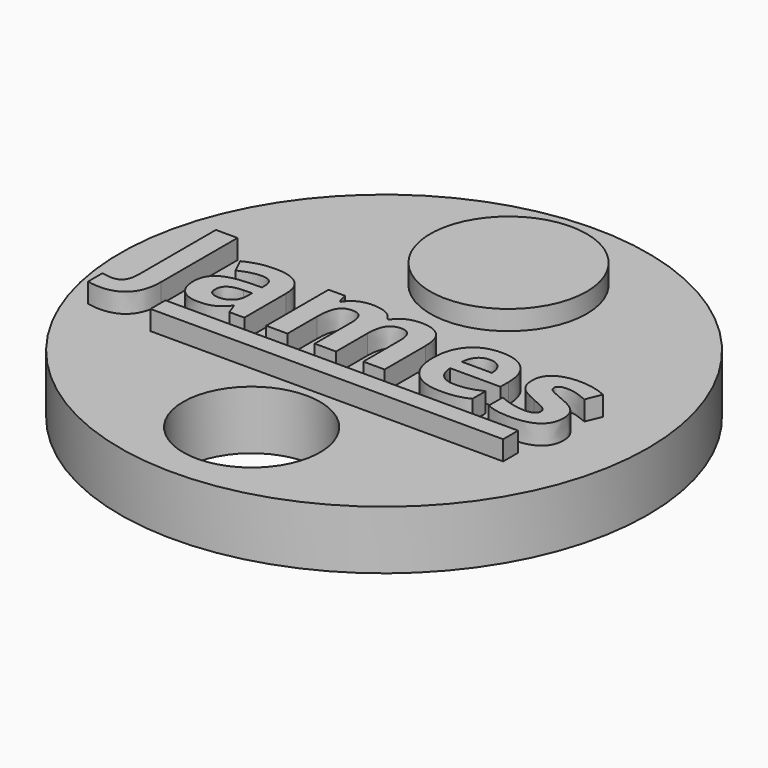
from build123d import *

# Parameters (mm, degrees)
F0_R         = 34.29
F1_DEPTH     = 7.62
F3_DEPTH     = 7.62
F4_TEXT_SIZE = 18.5547053762
F5_DEPTH     = 2.54
F6_R         = 10.16
F7_DEPTH     = 2.54
F10_D        = 15.24
F11_W        = 45.8176825196
F11_H        = 2.4243537337
F12_DEPTH    = 2.54
F15_D        = 17.78


# Not quite as in the source:
# - Text() gives the source's letters only with a copy of the font that has no kerning and outlines rounded to 1/6400 em; it was checked with that copy


with BuildPart() as f1:
    # F0 (on Top) → F1 (new body)
    with BuildSketch(Plane.XY):
        Circle(F0_R)
    extrude(amount=F1_DEPTH)

    # F4 (on face) → F5 (join)
    with BuildSketch(Plane.XY.offset(7.62)):
        with Locations((-28.5104531795, -7.0048975758)):
            Text('James', F4_TEXT_SIZE, font='Open Sans', font_style=FontStyle.BOLD, text_align=(TextAlign.LEFT, TextAlign.BOTTOM))
    extrude(amount=F5_DEPTH)

    # F6 (on face) → F7 (join)
    with BuildSketch(Plane.XY.offset(7.62)):
        with Locations((0.8362137014, 19.1624257714)):
            Circle(F6_R)
    extrude(amount=F7_DEPTH)

    # F11 (on face) → F12 (join)
    with BuildSketch(Plane.XY.offset(7.62)):
        with Locations((1.7281295732, -10.2478833869)):
            Rectangle(F11_W, F11_H)
    extrude(amount=F12_DEPTH)

    # F15 (through all)
    with Locations(Plane.XY.offset(7.62)):
        with Locations((0, -21.506447345)):
            Hole(F15_D / 2)


with BuildPart() as f3:
    # F2 (on face) → F3 (new body)
    with BuildSketch(Plane(origin=(0, 0, 0), x_dir=(1, 0, 0), z_dir=(0, 0, -1))):
        with BuildLine():
            ThreePointArc((12.5342215534, -31.9170391805), (-0.1799562098, -34.2895277856), (-12.8685320057, -31.7837219976))
            ThreePointArc((-12.8685320057, -31.7837219976), (-0.3185795997, -60.70334581), (12.5342215534, -31.9170391805))
        make_face()
    extrude(amount=-F3_DEPTH)

    # F10 (through all)
    with Locations(Plane.XY.offset(7.62)):
        with Locations((0, 49.184050411)):
            Hole(F10_D / 2)


solid = f1.part
